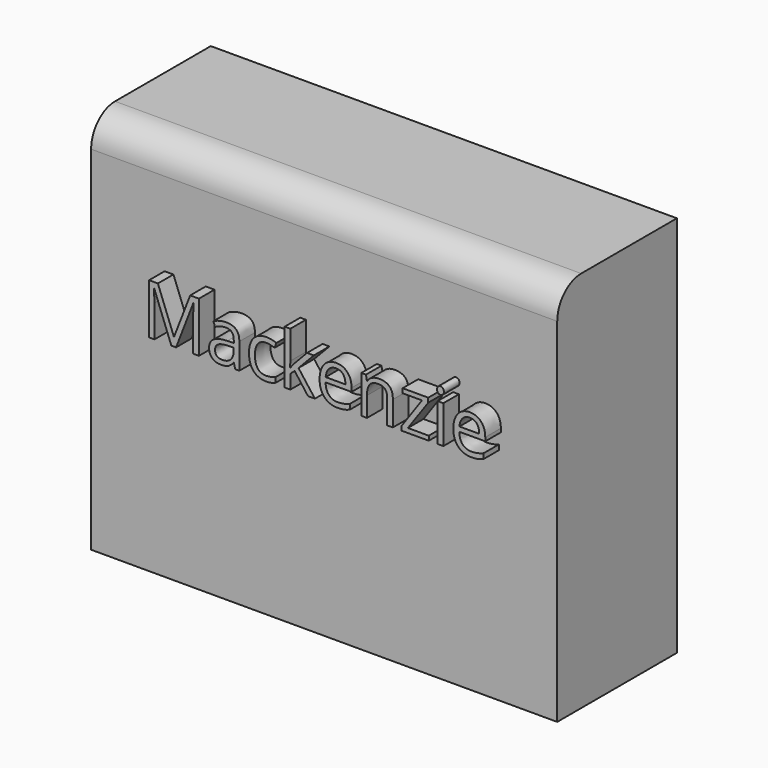
from build123d import *

# Parameters (mm, degrees)
F0_W         = 79.1588276625
F0_H         = 64.9726614356
F1_DEPTH     = 25.4
F2_R         = 5.08
F3_T         = -2.54
F4_TEXT_SIZE = 11.9797410055
F5_DEPTH     = 28.702


# Not quite as in the source:
# - Text() gives the source's letters only with a copy of the font that has no kerning and outlines rounded to 1/6400 em; it was checked with that copy


with BuildPart() as f1:
    # F0 (on Front) → F1 (new body)
    with BuildSketch(Plane.XZ):
        with Locations((-0.709310174, -4.965160042)):
            Rectangle(F0_W, F0_H)
    extrude(amount=F1_DEPTH)

    # F2
    f2_edges = [f1.edges().sort_by_distance(p)[0] for p in [
        (-0.70931, -25.4, 27.521171),
    ]]
    fillet(f2_edges, radius=F2_R)

    # F3
    f3_openings = [f1.faces().sort_by_distance(p)[0] for p in [
        (-0.70931, -12.7, -37.451491),
    ]]
    offset(amount=F3_T, openings=f3_openings)

    # F4 (on Front) → F5 (join)
    with BuildSketch(Plane.XZ):
        with Locations((-28.9811082184, -0.3064699704)):
            Text('Mackenzie', F4_TEXT_SIZE, font='Open Sans', text_align=(TextAlign.LEFT, TextAlign.BOTTOM))
    extrude(amount=F5_DEPTH)


solid = f1.part
